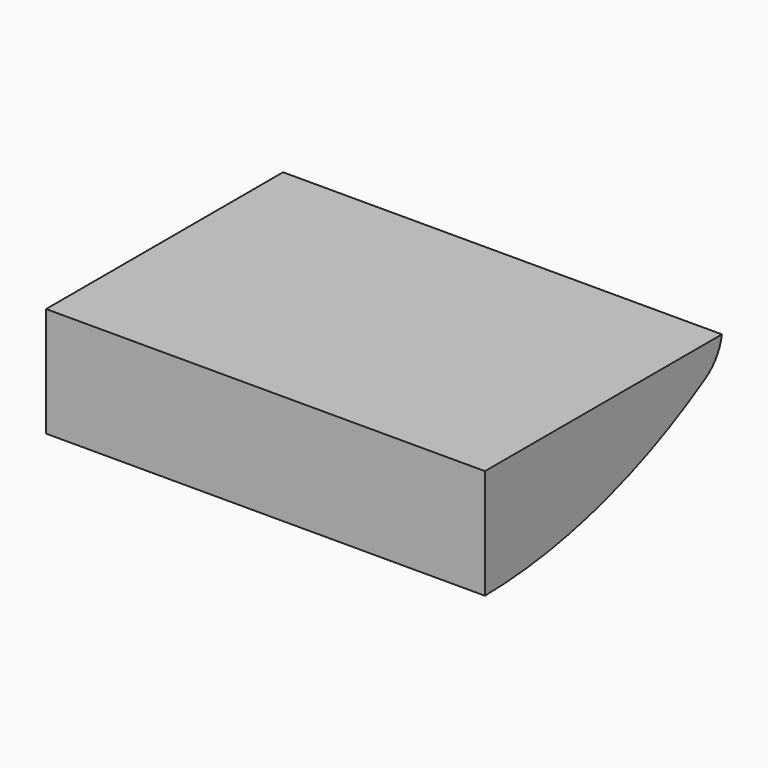
from build123d import *

# Parameters (mm, degrees)
F0_W        = 10
F0_H        = 7.142
F1_DEPTH    = 2.5
F3_DEPTH    = 10.001
F4_T1_DEPTH = 12.7651557864
F6_W        = 8
F6_H        = 0.5
F7_DEPTH    = 2


# Not quite as in the source:
# - a fillet or chamfer that OpenCascade refuses, or shapes differently, is made with other operations: its cross-section is extruded or revolved along the edge and cut away or added


with BuildPart() as f1:
    # F0 (on Top) → F1 (new body)
    with BuildSketch(Plane.XY):
        with Locations((5, 3.571)):
            Rectangle(F0_W, F0_H)
    extrude(amount=F1_DEPTH)

    # F2 (on face) → F3 (cut, through all)
    with BuildSketch(Plane(origin=(0, 0, 0), x_dir=(0, -1, 0), z_dir=(-1, 0, 0))):
        with BuildLine():
            ThreePointArc((0, 0), (-3.5295320322, 0.5584308586), (-6.75, 2.106987431))
            Line((-6.75, 2.106987431), (-6.75, 12.27143))
            Line((-6.75, 12.27143), (-9.8289949819, -2.3460234515))
            Line((-9.8289949819, -2.3460234515), (0, 0))
        make_face()
    extrude(amount=-F3_DEPTH, mode=Mode.SUBTRACT)

    # F4: fillet of radius 1 on 1 edges, made by hand

    # F4_s2 → F4_t1 (cut)
    with BuildSketch(Plane.YZ.offset(-1.3825778932)):
        with BuildLine():
            ThreePointArc((6.75, 2.5), (6.5929931831, 2.1031503004), (6.2848187014, 1.8079058028))
            ThreePointArc((6.2848187014, 1.8079058028), (6.5190889746, 1.9548341876), (6.75, 2.106987431))
            Line((6.75, 2.106987431), (6.75, 2.5))
        make_face()
    extrude(amount=F4_T1_DEPTH, mode=Mode.SUBTRACT)

    # F6 (on offset) → F7 (cut)
    with BuildSketch(Plane.XY):
        with Locations((5, 4.5299213873)):
            Rectangle(F6_W, F6_H)
        with Locations((5, 3.5299213873)):
            Rectangle(F6_W, F6_H)
        with Locations((5, 2.5299213873)):
            Rectangle(F6_W, F6_H)
        with Locations((5, 1.5299213873)):
            Rectangle(F6_W, F6_H)
        with Locations((5, 5.5299213873)):
            Rectangle(F6_W, F6_H)
    extrude(amount=F7_DEPTH, mode=Mode.SUBTRACT)


solid = f1.part
